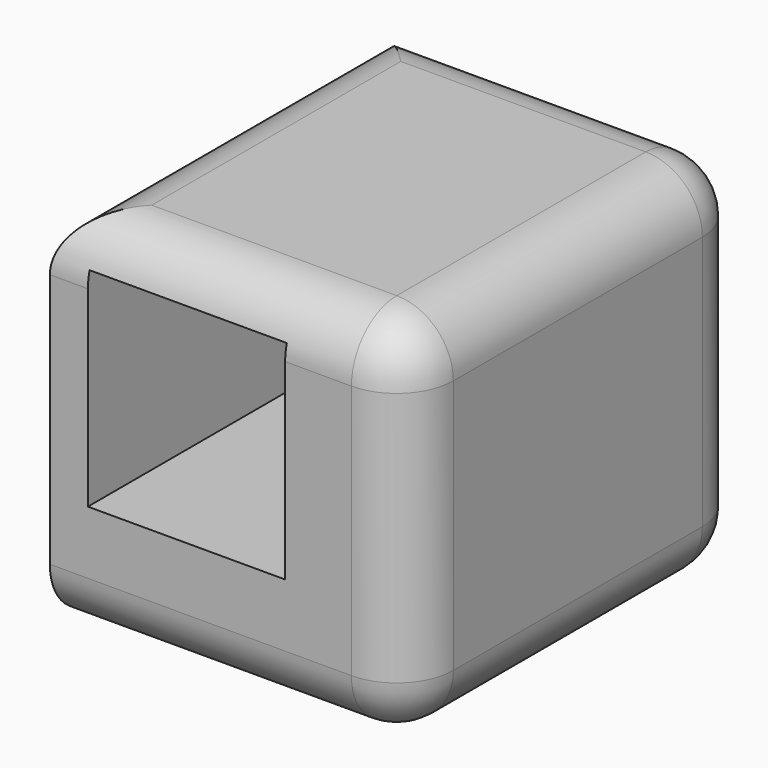
from build123d import *

# Parameters (mm, degrees)
F0_W         = 25.3122672439
F0_H         = 26.0148867965
F1_DEPTH     = 30
F2_W         = 13.9388088137
F2_H         = 14.6495383233
F3_DEPTH     = 32
F4_T1_DEPTH  = 18.0148867965
F4_T3_DEPTH  = 31.3122672439
F4_T5_DEPTH  = 36
F4_T7_DEPTH  = 22
F4_T9_DEPTH  = 50
F4_T11_DEPTH = 32.0148867965
F4_S15_W     = 4
F4_S15_H     = 4
F4_T16_DEPTH = 4
F4_S21_W     = 4
F4_S21_H     = 4
F4_T22_DEPTH = 4
F4_S27_W     = 4
F4_S27_H     = 4
F4_T28_DEPTH = 4
F5_T1_DEPTH  = 31.3122672439
F5_S5_W      = 4
F5_S5_H      = 4
F5_T6_DEPTH  = 4


# Not quite as in the source:
# - a fillet or chamfer that OpenCascade refuses, or shapes differently, is made with other operations: its cross-section is extruded or revolved along the edge and cut away or added


with BuildPart() as f1:
    # F0 (on Front) → F1 (new body)
    with BuildSketch(Plane.XZ):
        with Locations((12.6561336219, 13.0074433982)):
            Rectangle(F0_W, F0_H)
    extrude(amount=F1_DEPTH)

    # F2 (on face) → F3 (cut)
    with BuildSketch(Plane(origin=(0, 0, 0), x_dir=(-1, 0, 0), z_dir=(0, 1, 0))):
        with Locations((-9.6562495455, 15.7833071426)):
            Rectangle(F2_W, F2_H)
    extrude(amount=-F3_DEPTH, mode=Mode.SUBTRACT)

    # F4: fillet of radius 4 on 8 edges, made by hand

    # F4_s2 → F4_t1 (cut)
    with BuildSketch(Plane.XY.offset(4)):
        with BuildLine():
            ThreePointArc((21.3122672439, -30), (24.1406943686, -28.8284271247), (25.3122672439, -26))
            Line((25.3122672439, -26), (25.3122672439, -30))
            Line((25.3122672439, -30), (21.3122672439, -30))
        make_face()
    extrude(amount=F4_T1_DEPTH, mode=Mode.SUBTRACT)

    # F4_s4 → F4_t3 (cut)
    with BuildSketch(Plane.YZ.offset(-10)):
        with BuildLine():
            ThreePointArc((-26, 26.0148867965), (-28.8284271247, 24.8433139212), (-30, 22.0148867965))
            Line((-30, 22.0148867965), (-30, 26.0148867965))
            Line((-30, 26.0148867965), (-26, 26.0148867965))
        make_face()
        with BuildLine():
            ThreePointArc((-26, 0), (-28.8284271247, 1.1715728753), (-30, 4))
            Line((-30, 4), (-30, 0))
            Line((-30, 0), (-26, 0))
        make_face()
        with BuildLine():
            ThreePointArc((-4, 26.0148867965), (-1.1715728753, 24.8433139212), (0, 22.0148867965))
            Line((0, 22.0148867965), (0, 26.0148867965))
            Line((0, 26.0148867965), (-4, 26.0148867965))
        make_face()
    extrude(amount=F4_T3_DEPTH, mode=Mode.SUBTRACT)

    # F4_s6 → F4_t5 (cut)
    with BuildSketch(Plane.XZ.offset(-10)):
        with BuildLine():
            ThreePointArc((21.3122672439, 0), (24.1406943686, 1.1715728753), (25.3122672439, 4))
            Line((25.3122672439, 4), (25.3122672439, 0))
            Line((25.3122672439, 0), (21.3122672439, 0))
        make_face()
    extrude(amount=F4_T5_DEPTH, mode=Mode.SUBTRACT)

    # F4_s8 → F4_t7 (cut)
    with BuildSketch(Plane.XZ.offset(4)):
        with BuildLine():
            ThreePointArc((21.3122672439, 26.0148867965), (24.1406943686, 24.8433139212), (25.3122672439, 22.0148867965))
            Line((25.3122672439, 22.0148867965), (25.3122672439, 26.0148867965))
            Line((25.3122672439, 26.0148867965), (21.3122672439, 26.0148867965))
        make_face()
    extrude(amount=F4_T7_DEPTH, mode=Mode.SUBTRACT)

    # F4_s10 → F4_t9 (cut)
    with BuildSketch(Plane.XZ.offset(-10)):
        with BuildLine():
            ThreePointArc((0, 22.0148867965), (1.1715728753, 24.8433139212), (4, 26.0148867965))
            Line((4, 26.0148867965), (0, 26.0148867965))
            Line((0, 26.0148867965), (0, 22.0148867965))
        make_face()
    extrude(amount=F4_T9_DEPTH, mode=Mode.SUBTRACT)

    # F4_s12 → F4_t11 (cut)
    with BuildSketch(Plane.XY.offset(-10)):
        with BuildLine():
            ThreePointArc((21.3122672439, 0), (24.1406943686, -1.1715728753), (25.3122672439, -4))
            Line((25.3122672439, -4), (25.3122672439, 0))
            Line((25.3122672439, 0), (21.3122672439, 0))
        make_face()
    extrude(amount=F4_T11_DEPTH, mode=Mode.SUBTRACT)


with BuildPart() as f4_tool14:
    # F4_s15 → F4_t16 (new body)
    with BuildSketch(Plane.XY.offset(4)):
        with Locations((23.3122672439, -28)):
            Rectangle(F4_S15_W, F4_S15_H)
    extrude(amount=-F4_T16_DEPTH)

    # F4_s17 → F4_t18 (revolve, cut)
    with BuildSketch(Plane(origin=(21.3122672439, -26, 4), x_dir=(-0.7071067812, 0.7071067812, 0), z_dir=(-0.7071067812, -0.7071067812, 0))):
        with BuildLine():
            ThreePointArc((0, -4), (4, 0), (0, 4))
            Line((0, 4), (0, -4))
        make_face()
    revolve(axis=Axis((21.3122672439, -26, 4), (0, 0, -1)), mode=Mode.SUBTRACT)


with BuildPart() as f1_1:
    add(f1.part)

    # F4_t13: cut F4_tool14
    add(f4_tool14.part, mode=Mode.SUBTRACT)


with BuildPart() as f4_tool20:
    # F4_s21 → F4_t22 (new body)
    with BuildSketch(Plane.XY.offset(22.0148867965)):
        with Locations((23.3122672439, -28)):
            Rectangle(F4_S21_W, F4_S21_H)
    extrude(amount=F4_T22_DEPTH)

    # F4_s23 → F4_t24 (revolve, cut)
    with BuildSketch(Plane(origin=(21.3122672439, -26, 22.0148867965), x_dir=(-0.7071067812, 0.7071067812, 0), z_dir=(0.7071067812, 0.7071067812, 0))):
        with BuildLine():
            ThreePointArc((0, -4), (4, 0), (0, 4))
            Line((0, 4), (0, -4))
        make_face()
    revolve(axis=Axis((21.3122672439, -26, 22.0148867965), (0, 0, 1)), mode=Mode.SUBTRACT)


with BuildPart() as f1_2:
    add(f1_1.part)

    # F4_t19: cut F4_tool20
    add(f4_tool20.part, mode=Mode.SUBTRACT)


with BuildPart() as f4_tool26:
    # F4_s27 → F4_t28 (new body)
    with BuildSketch(Plane.XY.offset(22.0148867965)):
        with Locations((23.3122672439, -2)):
            Rectangle(F4_S27_W, F4_S27_H)
    extrude(amount=F4_T28_DEPTH)

    # F4_s29 → F4_t30 (revolve, cut)
    with BuildSketch(Plane(origin=(21.3122672439, -4, 22.0148867965), x_dir=(-0.7071067812, -0.7071067812, 0), z_dir=(-0.7071067812, 0.7071067812, 0))):
        with BuildLine():
            ThreePointArc((0, -4), (4, 0), (0, 4))
            Line((0, 4), (0, -4))
        make_face()
    revolve(axis=Axis((21.3122672439, -4, 22.0148867965), (0, 0, 1)), mode=Mode.SUBTRACT)


with BuildPart() as f1_3:
    add(f1_2.part)

    # F4_t25: cut F4_tool26
    add(f4_tool26.part, mode=Mode.SUBTRACT)

    # F5: fillet of radius 4 on 1 edges, made by hand

    # F5_s2 → F5_t1 (cut)
    with BuildSketch(Plane.YZ.offset(-10)):
        with BuildLine():
            ThreePointArc((0, 4), (-1.1715728753, 1.1715728753), (-4, 0))
            Line((-4, 0), (0, 0))
            Line((0, 0), (0, 4))
        make_face()
    extrude(amount=F5_T1_DEPTH, mode=Mode.SUBTRACT)


with BuildPart() as f5_tool4:
    # F5_s5 → F5_t6 (new body)
    with BuildSketch(Plane.XZ.offset(4)):
        with Locations((23.3122672439, 2)):
            Rectangle(F5_S5_W, F5_S5_H)
    extrude(amount=-F5_T6_DEPTH)

    # F5_s7 → F5_t8 (revolve, cut)
    with BuildSketch(Plane(origin=(21.3122672439, -4, 4), x_dir=(-0.7071067812, 0, 0.7071067812), z_dir=(-0.7071067812, 0, -0.7071067812))):
        with BuildLine():
            ThreePointArc((0, -4), (4, 0), (0, 4))
            Line((0, 4), (0, -4))
        make_face()
    revolve(axis=Axis((21.3122672439, -4, 4), (0, 1, 0)), mode=Mode.SUBTRACT)


with BuildPart() as f1_4:
    add(f1_3.part)

    # F5_t3: cut F5_tool4
    add(f5_tool4.part, mode=Mode.SUBTRACT)


solid = f1_4.part
